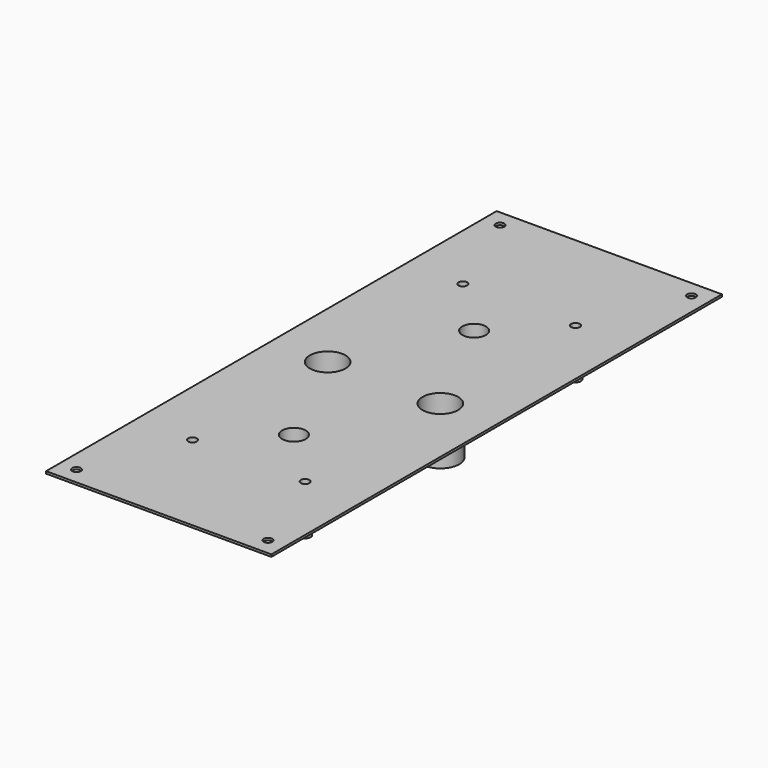
from build123d import *

# Parameters (mm, degrees)
F0_W     = 1000
F0_H     = 2500
F0_R     = 19.15
F0_R_2   = 52.15
F0_R_3   = 79.15
F1_DEPTH = 10
F2_R     = 24
F2_R_2   = 19.15
F2_R_3   = 57.15
F2_R_4   = 52.15
F2_R_5   = 84.15
F2_R_6   = 79.15
F3_DEPTH = 200


with BuildPart() as f1:
    # F0 (on Top) → F1 (new body)
    with BuildSketch(Plane.XY):
        Rectangle(F0_W, F0_H)
        with Locations((-425, -1175)):
            Circle(F0_R, mode=Mode.SUBTRACT)
        with Locations((-250, -750)):
            Circle(F0_R, mode=Mode.SUBTRACT)
        with Locations((425, -1175)):
            Circle(F0_R, mode=Mode.SUBTRACT)
        with Locations((250, -750)):
            Circle(F0_R, mode=Mode.SUBTRACT)
        with Locations((0, -500)):
            Circle(F0_R_2, mode=Mode.SUBTRACT)
        with Locations((-250, 0)):
            Circle(F0_R_3, mode=Mode.SUBTRACT)
        with Locations((-425, 1175)):
            Circle(F0_R, mode=Mode.SUBTRACT)
        with Locations((-250, 750)):
            Circle(F0_R, mode=Mode.SUBTRACT)
        with Locations((0, 500)):
            Circle(F0_R_2, mode=Mode.SUBTRACT)
        with Locations((250, 0)):
            Circle(F0_R_3, mode=Mode.SUBTRACT)
        with Locations((250, 750)):
            Circle(F0_R, mode=Mode.SUBTRACT)
        with Locations((425, 1175)):
            Circle(F0_R, mode=Mode.SUBTRACT)
    extrude(amount=F1_DEPTH)

    # F2 (on face) → F3 (join)
    with BuildSketch(Plane(origin=(0, 0, 0), x_dir=(1, 0, 0), z_dir=(0, 0, -1))):
        with Locations((250, 750)):
            Circle(F2_R)
        with Locations((250, 750)):
            Circle(F2_R_2, mode=Mode.SUBTRACT)
        with Locations((-250, 750)):
            Circle(F2_R)
        with Locations((-250, 750)):
            Circle(F2_R_2, mode=Mode.SUBTRACT)
        with Locations((0, 500)):
            Circle(F2_R_3)
        with Locations((0, 500)):
            Circle(F2_R_4, mode=Mode.SUBTRACT)
        with Locations((250, 0)):
            Circle(F2_R_5)
        with Locations((250, 0)):
            Circle(F2_R_6, mode=Mode.SUBTRACT)
        with Locations((0, -500)):
            Circle(F2_R_3)
        with Locations((0, -500)):
            Circle(F2_R_4, mode=Mode.SUBTRACT)
        with Locations((250, -750)):
            Circle(F2_R)
        with Locations((250, -750)):
            Circle(F2_R_2, mode=Mode.SUBTRACT)
        with Locations((-250, -750)):
            Circle(F2_R)
        with Locations((-250, -750)):
            Circle(F2_R_2, mode=Mode.SUBTRACT)
        with Locations((-250, 0)):
            Circle(F2_R_5)
        with Locations((-250, 0)):
            Circle(F2_R_6, mode=Mode.SUBTRACT)
    extrude(amount=F3_DEPTH)


solid = f1.part
